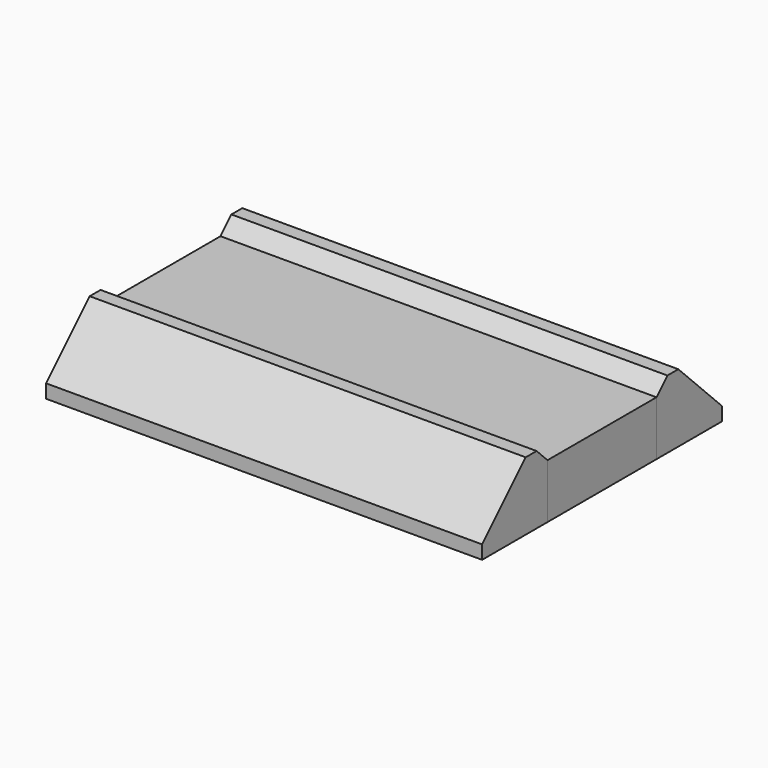
from build123d import *

# Parameters (mm, degrees)
F0_W      = 160
F0_H      = 5
F1_DEPTH  = 25
F0_H_2    = 50
F2_DEPTH  = 20
F3_SIZE   = 4.99999
F3_2_SIZE = 4.99999
F4_DEPTH  = 25
F5_DEPTH  = 25
F6_SIZE   = 20
F6_2_SIZE = 20


# Not quite as in the source:
# - a fillet or chamfer is up to 0.001 mm smaller than in the source, because OpenCascade refuses the exact size


with BuildPart() as f1:
    # F0 (on Top) → F1 (new body)
    with BuildSketch(Plane.XY):
        with Locations((2.5181677192, 6.6137810796)):
            Rectangle(F0_W, F0_H)
    extrude(amount=F1_DEPTH)

    # F3 (size 5 in the source; OpenCascade refuses exactly that, so slightly less here)
    f3_edges = [f1.edges().sort_by_distance(p)[0] for p in [
        (2.518168, 4.113781, 25),
    ]]
    chamfer(f3_edges, length=F3_SIZE)

    # F4 (add): a face of the model
    f4_faces = [f1.faces().sort_by_distance(p)[0] for p in [
        (2.5181677192, 9.1137810796, 12.5),
    ]]
    extrude(f4_faces, amount=F4_DEPTH)

    # F6
    f6_edges = [f1.edges().sort_by_distance(p)[0] for p in [
        (2.518168, 34.113781, 25),
    ]]
    chamfer(f6_edges, length=F6_SIZE)


with BuildPart() as f1b:
    # F0 (on Top) → F1, piece 2 (new body)
    with BuildSketch(Plane.XY):
        with Locations((2.5181677192, -48.3862189204)):
            Rectangle(F0_W, F0_H)
    extrude(amount=F1_DEPTH)

    # F3#2 (size 5 in the source; OpenCascade refuses exactly that, so slightly less here)
    f3_2_edges = [f1b.edges().sort_by_distance(p)[0] for p in [
        (2.518168, -45.886219, 25),
    ]]
    chamfer(f3_2_edges, length=F3_2_SIZE)

    # F5 (add): a face of the model
    f5_faces = [f1b.faces().sort_by_distance(p)[0] for p in [
        (2.5181677192, -50.8862189204, 12.5),
    ]]
    extrude(f5_faces, amount=F5_DEPTH)

    # F6#2
    f6_2_edges = [f1b.edges().sort_by_distance(p)[0] for p in [
        (2.518168, -75.886219, 25),
    ]]
    chamfer(f6_2_edges, length=F6_2_SIZE)


with BuildPart() as f2:
    # F0 (on Top) → F2 (new body)
    with BuildSketch(Plane.XY):
        with Locations((2.5181677192, -20.8862189204)):
            Rectangle(F0_W, F0_H_2)
    extrude(amount=F2_DEPTH)


solid = Compound([f1.part, f1b.part, f2.part])
